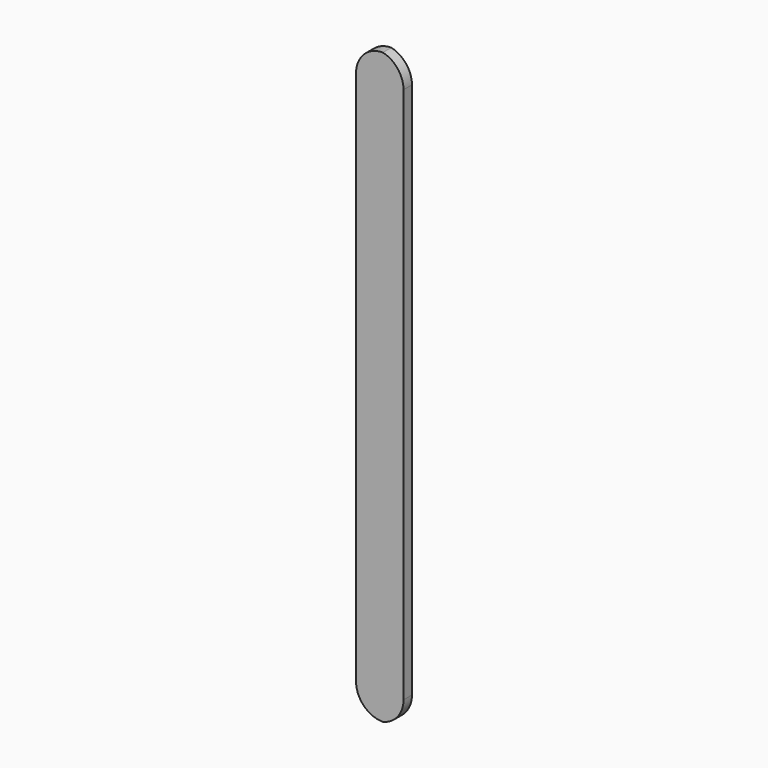
from build123d import *

# Parameters (mm, degrees)
F0_W        = 9
F0_H        = 111.76
F1_DEPTH    = 2
F2_R        = 5.08
F3_T1_DEPTH = 26.7289304257
F4_R        = 5.08
F5_T1_DEPTH = 26.7289304257


# Not quite as in the source:
# - a fillet or chamfer that OpenCascade refuses, or shapes differently, is made with other operations: its cross-section is extruded or revolved along the edge and cut away or added


with BuildPart() as f1:
    # F0 (on Front) → F1 (new body)
    with BuildSketch(Plane.XZ):
        with Locations((-4.5, 7.7518613339)):
            Rectangle(F0_W, F0_H)
    extrude(amount=F1_DEPTH)

    # F2
    f2_edges = [f1.edges().sort_by_distance(p)[0] for p in [
        (-9, -1, 63.631861),
    ]]
    fillet(f2_edges, radius=F2_R)

    # F3: fillet of radius 5.08 on 1 edges, made by hand

    # F3_s2 → F3_t1 (cut)
    with BuildSketch(Plane.XZ.offset(-12.3644652129)):
        with BuildLine():
            ThreePointArc((-3.92, 63.6318613339), (-1.0988443889, 61.8415149962), (0, 58.6860752487))
            Line((0, 58.6860752487), (0, 63.6318613339))
            Line((0, 63.6318613339), (-3.92, 63.6318613339))
        make_face()
    extrude(amount=F3_T1_DEPTH, mode=Mode.SUBTRACT)

    # F4
    f4_edges = [f1.edges().sort_by_distance(p)[0] for p in [
        (-9, -1, -48.128139),
    ]]
    fillet(f4_edges, radius=F4_R)

    # F5: fillet of radius 5.08 on 1 edges, made by hand

    # F5_s2 → F5_t1 (cut)
    with BuildSketch(Plane.XZ.offset(-12.3644652129)):
        with BuildLine():
            ThreePointArc((-3.92, -48.1281386661), (-1.0988443889, -46.3377923285), (0, -43.182352581))
            Line((0, -43.182352581), (0, -48.1281386661))
            Line((0, -48.1281386661), (-3.92, -48.1281386661))
        make_face()
    extrude(amount=F5_T1_DEPTH, mode=Mode.SUBTRACT)


solid = f1.part
